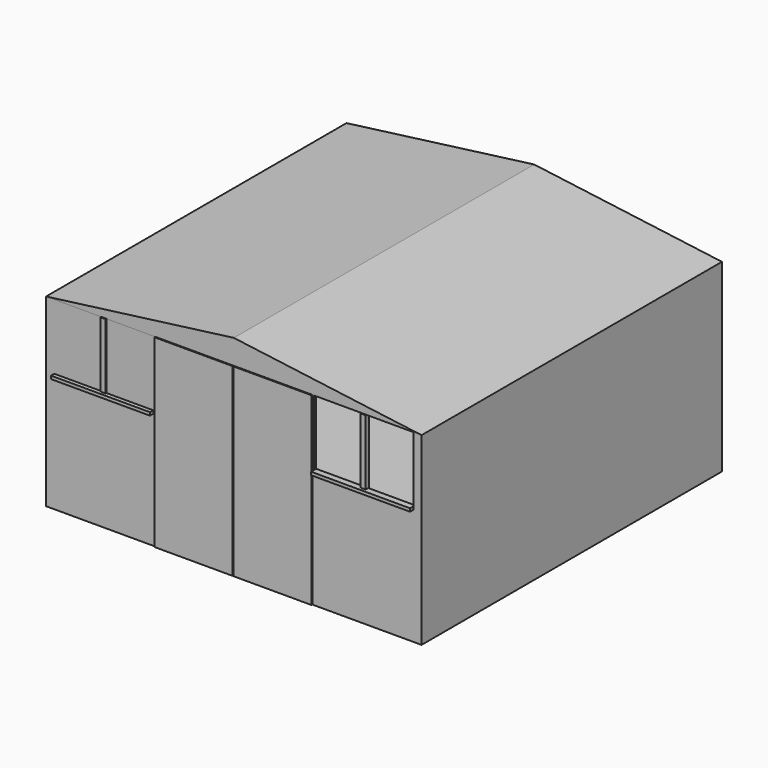
from build123d import *

# Parameters (mm, degrees)
F0_W          = 366
F0_H          = 366
F0_W_2        = 361.6
F0_H_2        = 361.6
F1_DEPTH      = 180
F2_DEPTH      = 2.2
F3_W          = 76
F3_H          = 180
F3_W_2        = 5
F3_H_2        = 63.7124854326
F4_DEPTH      = 1
F4_DEPTH_BACK = 3.3
F3_W_3        = 45.75
F5_DEPTH      = 25
F6_DEPTH      = 8
F7_DEPTH      = 4
F9_DEPTH      = 366


# Not quite as in the source:
# - a feature names something its author has since deleted; it is built from what else it names


with BuildPart() as f1:
    # F0 (on Top) → F1 (new body)
    with BuildSketch(Plane.XY):
        with Locations((183, -183)):
            Rectangle(F0_W, F0_H)
        with Locations((183, -183)):
            Rectangle(F0_W_2, F0_H_2, mode=Mode.SUBTRACT)
    extrude(amount=F1_DEPTH)

    # F0 (on Top) → F2 (join)
    with BuildSketch(Plane.XY):
        with Locations((183, -183)):
            Rectangle(F0_W_2, F0_H_2)
    extrude(amount=F2_DEPTH)

    # F3 (on face) → F4 (join, two sides)
    with BuildSketch(Plane.XZ.offset(366)) as f4_sk:
        with Locations((144.5, 90)):
            Rectangle(F3_W, F3_H)
        with Locations((221.5, 90)):
            Rectangle(F3_W, F3_H)
        with Locations((56.25, 148.1437572837)):
            Rectangle(F3_W_2, F3_H_2)
        with Locations((309.75, 148.1437572837)):
            Rectangle(F3_W_2, F3_H_2)
    extrude(amount=F4_DEPTH)
    extrude(f4_sk.sketch, amount=-F4_DEPTH_BACK)

    # F3 (on face) → F5 (cut)
    with BuildSketch(Plane.XZ.offset(366)):
        Polygon((104.5, 180), (106.5, 180), (182.5, 180), (183.5, 180), (259.5, 180), (261.5, 180), (307.25, 180), (312.25, 180), (358, 180), (366, 180), (183, 204), (0, 180), (8, 180), (53.75, 180), (58.75, 180), align=None)
        with Locations((284.375, 148.1437572837)):
            Rectangle(F3_W_3, F3_H_2)
        with Locations((335.125, 148.1437572837)):
            Rectangle(F3_W_3, F3_H_2)
    extrude(amount=-F5_DEPTH, mode=Mode.SUBTRACT)

    # F3 (on face) → F6 (join)
    with BuildSketch(Plane.XZ.offset(366)):
        Polygon((104.5, 180), (106.5, 180), (182.5, 180), (183.5, 180), (259.5, 180), (261.5, 180), (307.25, 180), (312.25, 180), (358, 180), (366, 180), (183, 204), (0, 180), (8, 180), (53.75, 180), (58.75, 180), align=None)
    extrude(amount=-F6_DEPTH)

    # F3 (on face) → F7 (join)
    with BuildSketch(Plane.XZ.offset(366)):
        Polygon((307.25, 116.2875145674), (261.5, 116.2875145674), (261.5, 113.2875145674), (358, 113.2875145674), (358, 116.2875145674), (312.25, 116.2875145674), align=None)
        Polygon((104.5, 113.2875145674), (104.5, 116.2875145674), (58.75, 116.2875145674), (53.75, 116.2875145674), (8, 116.2875145674), (8, 113.2875145674), align=None)
    extrude(amount=F7_DEPTH)


with BuildPart() as f9:
    # F8 (on face) → F9 (new body)
    with BuildSketch(Plane(origin=(0, 0, 0), x_dir=(-1, 0, 0), z_dir=(0, 1, 0))):
        Polygon((-183, 204), (-366, 180), (0, 180), align=None)
    extrude(amount=-F9_DEPTH)


solid = Compound([f1.part, f9.part])
